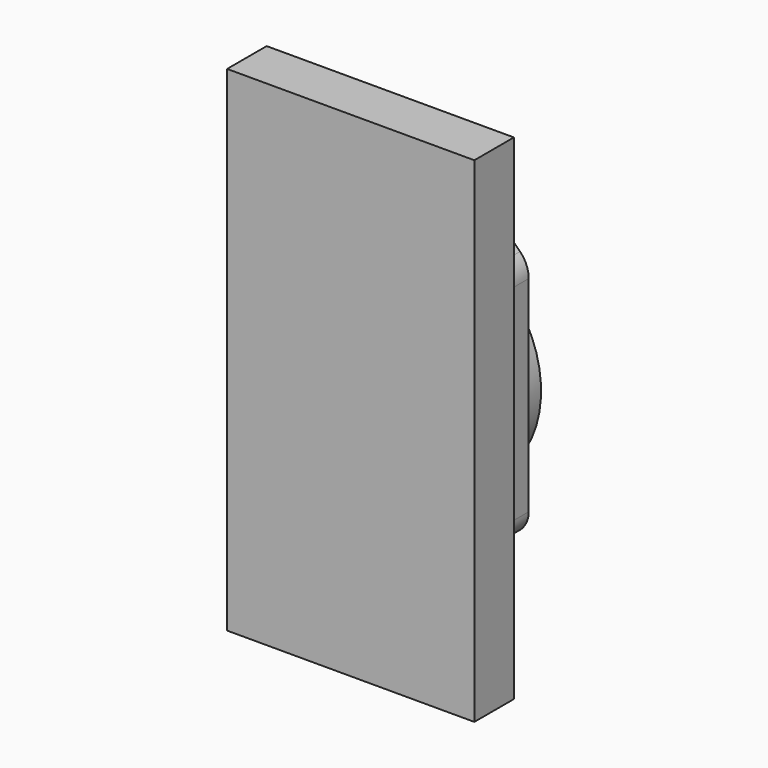
from build123d import *

# Parameters (mm, degrees)
F0_W      = 100
F0_H      = 200
F1_DEPTH  = 20
F3_DEPTH  = 10
F5_DEPTH  = 10
F6_R      = 45
F6_R_2    = 30
F7_DEPTH  = 10
F8_R      = 30
F9_DEPTH  = 32
F11_D     = 10
F11_DEPTH = 15
F11_TIP   = 3.0043030951


with BuildPart() as f1:
    # F0 (on Front) → F1 (new body)
    with BuildSketch(Plane.XZ):
        Rectangle(F0_W, F0_H)
    extrude(amount=F1_DEPTH)

    # F2 (on face) → F3 (cut)
    with BuildSketch(Plane(origin=(0, 0, 0), x_dir=(-1, 0, 0), z_dir=(0, 1, 0))):
        with BuildLine():
            ThreePointArc((-28, -60), (-36.4852813742, -63.5147186258), (-40, -72))
            Line((-40, -72), (-40, -78))
            ThreePointArc((-40, -78), (-36.4852813742, -86.4852813742), (-28, -90))
            Line((-28, -90), (28, -90))
            ThreePointArc((28, -90), (36.4852813742, -86.4852813742), (40, -78))
            Line((40, -78), (40, -72))
            ThreePointArc((40, -72), (36.4852813742, -63.5147186258), (28, -60))
            Line((28, -60), (-28, -60))
        make_face()
    extrude(amount=-F3_DEPTH, mode=Mode.SUBTRACT)

    # F4 (on face) → F5 (join)
    with BuildSketch(Plane(origin=(0, 0, 0), x_dir=(-1, 0, 0), z_dir=(0, 1, 0))):
        with BuildLine():
            Line((-48, 45.029), (-48, -38))
            ThreePointArc((-48, -38), (-45.0710678119, -45.0710678119), (-38, -48))
            Line((-38, -48), (38, -48))
            ThreePointArc((38, -48), (45.0710678119, -45.0710678119), (48, -38))
            Line((48, -38), (48, 45.029))
            ThreePointArc((48, 45.029), (47.0866406093, 49.6209930314), (44.4856, 53.5139627365))
            Line((44.4856, 53.5139627365), (10.607, 87.3951071902))
            ThreePointArc((10.607, 87.3951071902), (0, 91.7889037696), (-10.607, 87.3951071902))
            Line((-10.607, 87.3951071902), (-44.4856, 53.5139627365))
            ThreePointArc((-44.4856, 53.5139627365), (-47.0866406093, 49.6209930314), (-48, 45.029))
        make_face()
    extrude(amount=F5_DEPTH)

    # F6 (on face) → F7 (join)
    with BuildSketch(Plane(origin=(0, 10, 0), x_dir=(-1, 0, 0), z_dir=(0, 1, 0))):
        Circle(F6_R)
        Circle(F6_R_2, mode=Mode.SUBTRACT)
        Circle(F6_R_2)
    extrude(amount=F7_DEPTH)

    # F8 (on face) → F9 (cut)
    with BuildSketch(Plane(origin=(0, 20, 0), x_dir=(-1, 0, 0), z_dir=(0, 1, 0))):
        Circle(F8_R)
    extrude(amount=-F9_DEPTH, mode=Mode.SUBTRACT)

    # F11
    with Locations(Plane(origin=(0, 20, 0), x_dir=(-1, 0, 0), z_dir=(0, 1, 0))):
        with Locations((-37.5, 0), (0, 37.5), (0, -37.5), (37.5, 0)):
            Hole(F11_D / 2, depth=F11_DEPTH)
            with Locations((0, 0, -(F11_DEPTH + F11_TIP / 2))):  # 118° drill point
                Cone(0, F11_D / 2, F11_TIP, mode=Mode.SUBTRACT)


solid = f1.part
